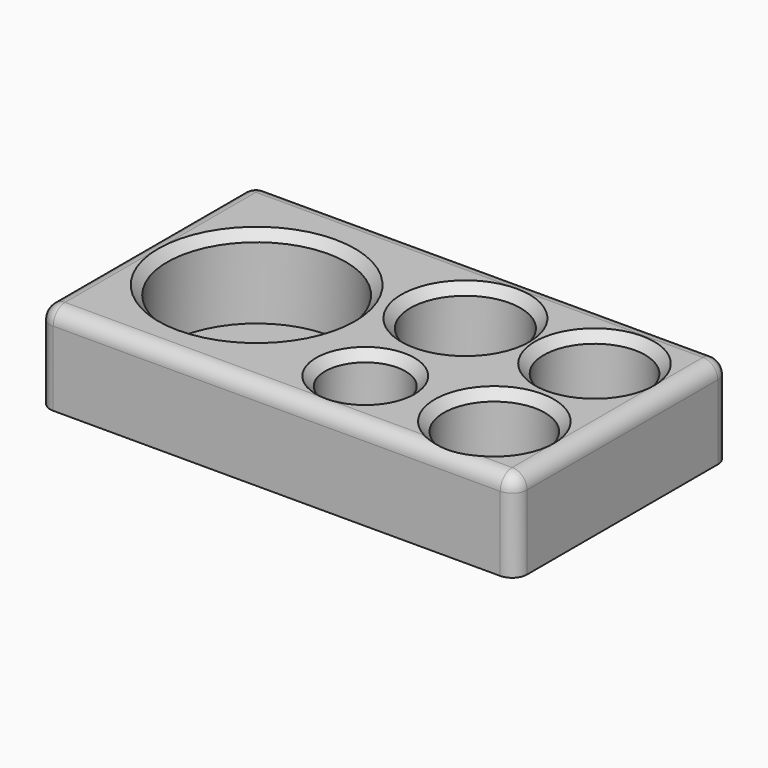
from build123d import *

# Parameters (mm, degrees)
F0_W     = 160
F0_H     = 90
F0_R     = 30
F0_R_2   = 13.5
F0_R_3   = 17
F0_R_4   = 18.5
F1_DEPTH = 30
F2_DEPTH = 3
F3_R     = 5
F4_R     = 5


# Not quite as in the source:
# - a fillet or chamfer that OpenCascade refuses, or shapes differently, is made with other operations: its cross-section is extruded or revolved along the edge and cut away or added


with BuildPart() as f1:
    # F0 (on Top) → F1 (new body)
    with BuildSketch(Plane.XY):
        with Locations((-52.1784374716, 16.3527858257)):
            Rectangle(F0_W, F0_H)
        with Locations((-94.1784374716, 15.4254203662)):
            Circle(F0_R, mode=Mode.SUBTRACT)
        with Locations((-39.6653786302, -7.1472141743)):
            Circle(F0_R_2, mode=Mode.SUBTRACT)
        with Locations((2.8215625284, -6.1201333007)):
            Circle(F0_R_3, mode=Mode.SUBTRACT)
        with Locations((-39.6653786302, 34.8527858257)):
            Circle(F0_R_4, mode=Mode.SUBTRACT)
        with Locations((2.8215625284, 35.9062709907)):
            Circle(F0_R_3, mode=Mode.SUBTRACT)
    extrude(amount=F1_DEPTH)

    # F0 (on Top) → F2 (join)
    with BuildSketch(Plane.XY):
        with Locations((-52.1784374716, 16.3527858257)):
            Rectangle(F0_W, F0_H)
        with Locations((-94.1784374716, 15.4254203662)):
            Circle(F0_R, mode=Mode.SUBTRACT)
        with Locations((-39.6653786302, -7.1472141743)):
            Circle(F0_R_2, mode=Mode.SUBTRACT)
        with Locations((2.8215625284, -6.1201333007)):
            Circle(F0_R_3, mode=Mode.SUBTRACT)
        with Locations((-39.6653786302, 34.8527858257)):
            Circle(F0_R_4, mode=Mode.SUBTRACT)
        with Locations((2.8215625284, 35.9062709907)):
            Circle(F0_R_3, mode=Mode.SUBTRACT)
        with Locations((-94.1784374716, 15.4254203662)):
            Circle(F0_R)
        with Locations((-39.6653786302, -7.1472141743)):
            Circle(F0_R_2)
        with Locations((2.8215625284, -6.1201333007)):
            Circle(F0_R_3)
        with Locations((2.8215625284, 35.9062709907)):
            Circle(F0_R_3)
        with Locations((-39.6653786302, 34.8527858257)):
            Circle(F0_R_4)
    extrude(amount=F2_DEPTH)

    # F3
    f3_edges = [f1.edges().sort_by_distance(p)[0] for p in [
        (27.821563, 61.352786, 15),
        (27.821563, -28.647214, 15),
        (-132.178437, -28.647214, 15),
        (-132.178437, 61.352786, 15),
    ]]
    fillet(f3_edges, radius=F3_R)

    # F4
    f4_edges = [f1.edges().sort_by_distance(p)[0] for p in [
        (-52.178437, 61.352786, 30),
        (27.821563, 16.352786, 30),
        (-52.178437, -28.647214, 30),
        (-132.178437, 16.352786, 30),
        (26.357096, -27.182748, 30),
        (26.357096, 59.88832, 30),
        (-130.713971, -27.182748, 30),
        (-130.713971, 59.88832, 30),
    ]]
    fillet(f4_edges, radius=F4_R)

    # F5: chamfer of 3 on 5 edges, made by hand

    # F5_s1 → F5_t2 (revolve, cut)
    with BuildSketch(Plane.XZ.offset(-15.4254203662)):
        Polygon((-61.1784374716, 30), (-64.1784374716, 27), (-64.1784374716, 30), align=None)
    revolve(axis=Axis((-94.1784374716, 15.4254203662, 30), (0, 0, 1)), mode=Mode.SUBTRACT)

    # F5_s3 → F5_t4 (revolve, cut)
    with BuildSketch(Plane.XZ.offset(-34.8527858257)):
        Polygon((-18.1653786302, 30), (-21.1653786302, 27), (-21.1653786302, 30), align=None)
    revolve(axis=Axis((-39.6653786302, 34.8527858257, 30), (0, 0, 1)), mode=Mode.SUBTRACT)

    # F5_s5 → F5_t6 (revolve, cut)
    with BuildSketch(Plane.XZ.offset(-35.9062709907)):
        Polygon((22.8215625284, 30), (19.8215625284, 27), (19.8215625284, 30), align=None)
    revolve(axis=Axis((2.8215625284, 35.9062709907, 30), (0, 0, 1)), mode=Mode.SUBTRACT)

    # F5_s7 → F5_t8 (revolve, cut)
    with BuildSketch(Plane.XZ.offset(6.1201333007)):
        Polygon((22.8215625284, 30), (19.8215625284, 27), (19.8215625284, 30), align=None)
    revolve(axis=Axis((2.8215625284, -6.1201333007, 30), (0, 0, 1)), mode=Mode.SUBTRACT)

    # F5_s9 → F5_t10 (revolve, cut)
    with BuildSketch(Plane.XZ.offset(7.1472141743)):
        Polygon((-23.1653786302, 30), (-26.1653786302, 27), (-26.1653786302, 30), align=None)
    revolve(axis=Axis((-39.6653786302, -7.1472141743, 30), (0, 0, 1)), mode=Mode.SUBTRACT)


solid = f1.part
